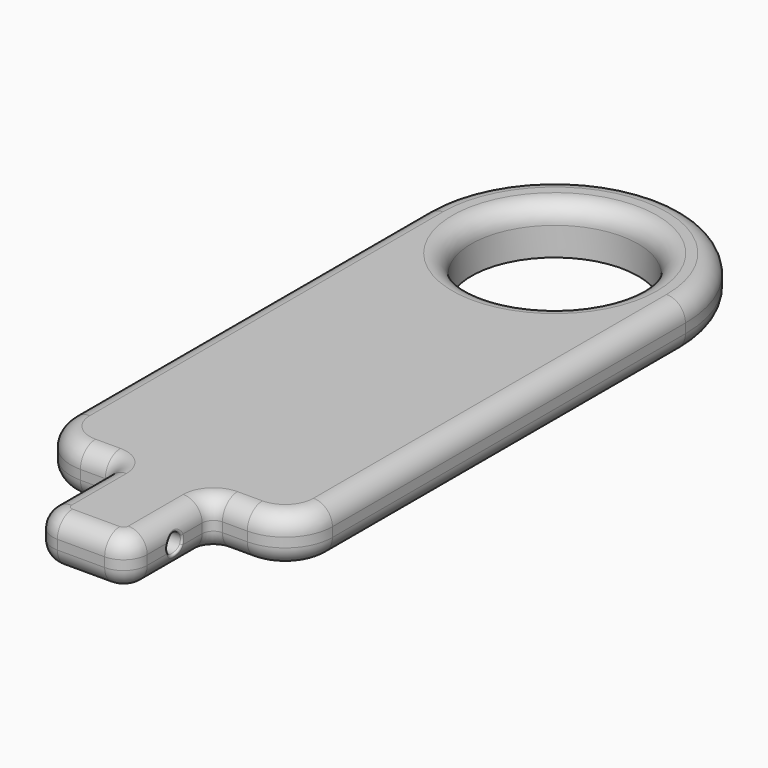
from build123d import *

# Parameters (mm, degrees)
F1_DEPTH = 12.7
F2_R     = 22.4175504924
F3_DEPTH = 12.7
F4_R     = 5.08
F5_R     = 2.54
F6_DEPTH = 25.4
F7_R     = 0.508


with BuildPart() as f1:
    # F0 (on Top) → F1 (new body)
    with BuildSketch(Plane.XY):
        with BuildLine():
            ThreePointArc((35.1175504924, 65.6300778079), (0, 100.7476283003), (-35.1175504924, 65.6300778079))
            Line((-35.1175504924, 65.6300778079), (35.1175504924, 65.6300778079))
        make_face()
        with BuildLine():
            Line((35.1175504924, 65.6300778079), (-35.1175504924, 65.6300778079))
            ThreePointArc((-35.1175504924, 65.6300778079), (0, 30.5125273154), (35.1175504924, 65.6300778079))
        make_face()
        with BuildLine():
            ThreePointArc((35.1175504924, 65.6300778079), (0, 30.5125273154), (-35.1175504924, 65.6300778079))
            Line((-35.1175504924, 65.6300778079), (-35.1175504924, -52.9300778079))
            ThreePointArc((-35.1175504924, -52.9300778079), (-31.3978066135, -61.9103339289), (-22.4175504924, -65.6300778079))
            Line((-22.4175504924, -65.6300778079), (-15.7272638846, -65.6300778079))
            ThreePointArc((-15.7272638846, -65.6300778079), (-13.5866650633, -66.5167428712), (-12.7, -68.6573416924))
            Line((-12.7, -68.6573416924), (-12.7, -87.1002871167))
            ThreePointArc((-12.7, -87.1002871167), (-10.8401280605, -91.5904151773), (-6.35, -93.4502871167))
            Line((-6.35, -93.4502871167), (6.35, -93.4502871167))
            ThreePointArc((6.35, -93.4502871167), (10.8401280605, -91.5904151773), (12.7, -87.1002871167))
            Line((12.7, -87.1002871167), (12.7, -68.6573416924))
            ThreePointArc((12.7, -68.6573416924), (13.5866650633, -66.5167428712), (15.7272638846, -65.6300778079))
            Line((15.7272638846, -65.6300778079), (22.4175504924, -65.6300778079))
            ThreePointArc((22.4175504924, -65.6300778079), (31.3978066135, -61.9103339289), (35.1175504924, -52.9300778079))
            Line((35.1175504924, -52.9300778079), (35.1175504924, 65.6300778079))
        make_face()
    extrude(amount=F1_DEPTH)

    # F2 (on face) → F3 (cut, through all)
    with BuildSketch(Plane.XY.offset(12.7)):
        with Locations((0, 65.6300778079)):
            Circle(F2_R)
    extrude(amount=-F3_DEPTH, mode=Mode.SUBTRACT)

    # F4
    f4_edges = [f1.edges().sort_by_distance(p)[0] for p in [
        (35.11755, 6.35, 12.7),
        (0, 100.747628, 0),
        (-22.41755, 65.630078, 12.7),
    ]]
    fillet(f4_edges, radius=F4_R)

    # F5 (on face) → F6 (cut, through all)
    with BuildSketch(Plane.YZ.offset(12.7)):
        with Locations((-77.8788144046, 6.35)):
            Circle(F5_R)
    extrude(amount=-F6_DEPTH, mode=Mode.SUBTRACT)

    # F7
    f7_edges = [f1.edges().sort_by_distance(p)[0] for p in [
        (12.7, -80.418814, 6.35),
        (12.7, -75.425363, 7.0074),
        (12.7, -75.425363, 5.6926),
        (12.538689, -77.878814, 8.89),
        (12.538689, -77.878814, 3.81),
        (-12.538689, -77.878814, 8.89),
        (-12.7, -75.425363, 5.6926),
        (-12.7, -80.418814, 6.35),
        (-12.7, -75.425363, 7.0074),
    ]]
    fillet(f7_edges, radius=F7_R)


solid = f1.part
